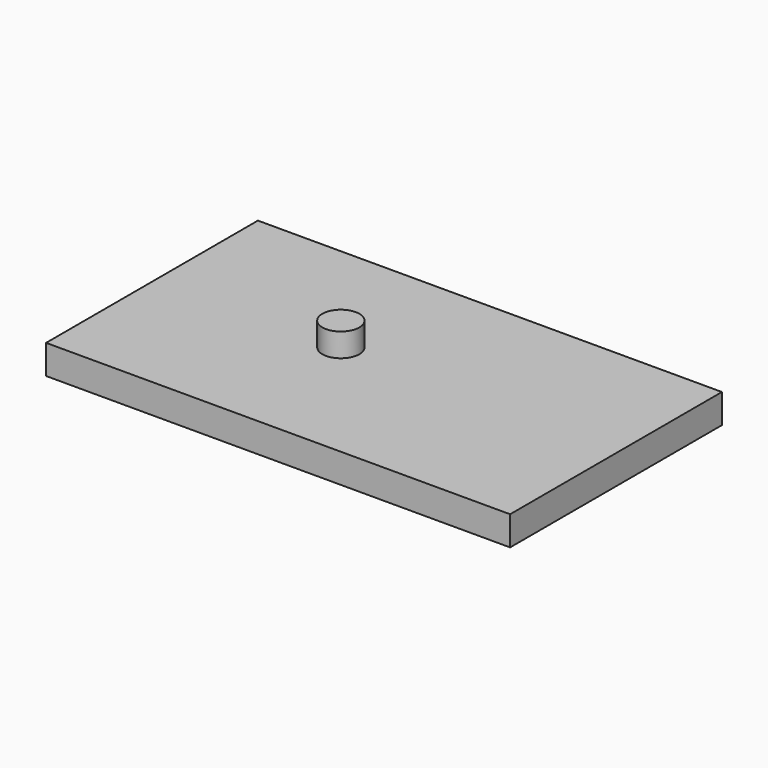
from build123d import *

# Parameters (mm, degrees)
F0_W     = 85.5915052816
F0_H     = 9.4415829517
F1_DEPTH = 150
F2_DEPTH = 150
F4_R     = 5.981115506
F5_DEPTH = 7.62


# Not quite as in the source:
# - a feature of the source that left no trace in its solid (it failed there, or was rolled back) is left out


with BuildPart() as f1:
    # F0 (on Right) → F1 (new body)
    with BuildSketch(Plane.YZ):
        with Locations((-29.4651468284, 4.7207914758)):
            Rectangle(F0_W, F0_H)
    extrude(amount=F1_DEPTH)

    # F2 (cut): a face of the model
    f2_faces = [f1.faces().sort_by_distance(p)[0] for p in [
        (75, -72.2608994693, 4.7207914758),
    ]]
    extrude(f2_faces, amount=F2_DEPTH, mode=Mode.SUBTRACT)

    # F4 (on face) → F5 (join)
    with BuildSketch(Plane.XY.offset(9.4415829517)):
        with Locations((59.6557557583, -27.7189966291)):
            Circle(F4_R)
    extrude(amount=F5_DEPTH)


solid = f1.part
